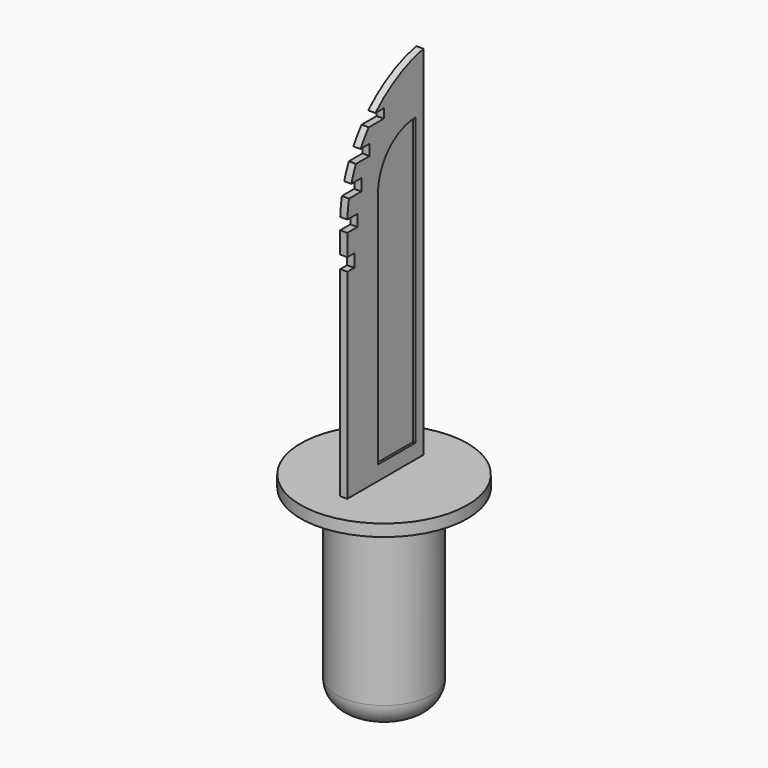
from build123d import *

# Parameters (mm, degrees)
F0_R        = 2
F1_DEPTH    = 8
F2_R        = 3.5
F2_R_2      = 2
F3_DEPTH    = 0.5
F4_W        = 0.3
F4_H        = 3.9893038338
F5_DEPTH    = 15
F6_T1_DEPTH = 24.7839198555
F7_R        = 1
F8_W        = 1.6560796648
F8_H        = 0.4959646612
F8_W_2      = 1.2781426776
F8_H_2      = 0.4874281585
F8_W_3      = 1.2889747159
F8_H_3      = 0.4549305886
F8_W_4      = 0.7887214828
F8_H_4      = 0.3866125997
F8_W_5      = 1.2771316105
F8_H_5      = 0.5377400666
F9_DEPTH    = 0.3
F11_DEPTH   = 0.1
F13_DEPTH   = 0.1


# Not quite as in the source:
# - a fillet or chamfer that OpenCascade refuses, or shapes differently, is made with other operations: its cross-section is extruded or revolved along the edge and cut away or added


with BuildPart() as f1:
    # F0 (on Top) → F1 (new body)
    with BuildSketch(Plane.XY):
        Circle(F0_R)
    extrude(amount=F1_DEPTH)

    # F2 (on face) → F3 (join)
    with BuildSketch(Plane.XY.offset(8)):
        Circle(F2_R)
        Circle(F2_R_2, mode=Mode.SUBTRACT)
        Circle(F2_R_2)
    extrude(amount=F3_DEPTH)

    # F4 (on face) → F5 (join)
    with BuildSketch(Plane.XY.offset(8.5)):
        with Locations((0, -0.1216841047)):
            Rectangle(F4_W, F4_H)
    extrude(amount=F5_DEPTH)

    # F6: fillet of radius 5 on 1 edges, made by hand

    # F6_s2 → F6_t1 (cut)
    with BuildSketch(Plane.YZ.offset(-12.3919599278)):
        with BuildLine():
            ThreePointArc((-2.1163360216, 18.6032160289), (-0.9927700034, 21.7612628279), (1.8729678122, 23.5))
            Line((1.8729678122, 23.5), (-2.1163360216, 23.5))
            Line((-2.1163360216, 23.5), (-2.1163360216, 18.6032160289))
        make_face()
    extrude(amount=F6_T1_DEPTH, mode=Mode.SUBTRACT)

    # F7
    f7_edges = [f1.edges().sort_by_distance(p)[0] for p in [
        (-2, 0, 0),
    ]]
    fillet(f7_edges, radius=F7_R)

    # F8 (on face) → F9 (cut)
    with BuildSketch(Plane(origin=(-0.15, 0, 0), x_dir=(0, -1, 0), z_dir=(-1, 0, 0))):
        with Locations((2.2049986292, 19.7972180322)):
            Rectangle(F8_W, F8_H)
        with Locations((2.2229513852, 18.5654982924)):
            Rectangle(F8_W_2, F8_H_2)
        with Locations((1.5892958909, 20.9105657414)):
            Rectangle(F8_W_3, F8_H_3)
        with Locations((0.598409262, 21.9545691277)):
            Rectangle(F8_W_4, F8_H_4)
        with Locations((2.3904092959, 17.1525618061)):
            Rectangle(F8_W_5, F8_H_5)
    extrude(amount=-F9_DEPTH, mode=Mode.SUBTRACT)

    # F10 (on face) → F11 (cut)
    with BuildSketch(Plane(origin=(-0.15, 0, 0), x_dir=(0, -1, 0), z_dir=(-1, 0, 0))):
        with BuildLine():
            Line((-1.4041818934, 21.1293072328), (-1.4041818934, 9.1293072328))
            Line((-1.4041818934, 9.1293072328), (0.5958181066, 9.1293072328))
            Line((0.5958181066, 9.1293072328), (0.5958181066, 19.1293072328))
            ThreePointArc((0.5958181066, 19.1293072328), (0.010031669, 20.5435207952), (-1.4041818934, 21.1293072328))
        make_face()
    extrude(amount=-F11_DEPTH, mode=Mode.SUBTRACT)

    # F12 (on face) → F13 (cut)
    with BuildSketch(Plane.YZ.offset(0.15)):
        with BuildLine():
            Line((-0.5063290591, 9.1143995523), (1.4634948457, 9.1143995523))
            Line((1.4634948457, 9.1143995523), (1.4634948457, 21.1303744976))
            ThreePointArc((1.4634948457, 21.1303744976), (0.06882846, 20.5341063118), (-0.5063290591, 19.1306021597))
            Line((-0.5063290591, 19.1306021597), (-0.5063290591, 9.1143995523))
        make_face()
    extrude(amount=-F13_DEPTH, mode=Mode.SUBTRACT)


solid = f1.part
